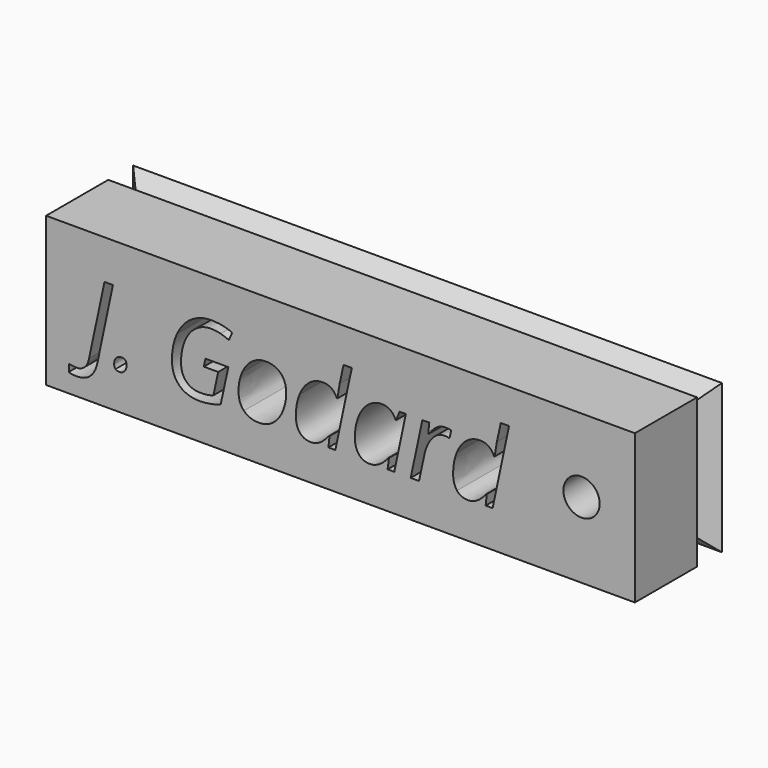
from build123d import *

# Parameters (mm, degrees)
F0_W        = 96.2526388466
F0_H        = 24.3639480323
F0_R        = 2.9624305705
F1_DEPTH    = 5.08
F2_T1_DEPTH = 50.49224719
F2_T3_DEPTH = 122.3809380044
F3_DEPTH    = 12.7


# Not quite as in the source:
# - a fillet or chamfer that OpenCascade refuses, or shapes differently, is made with other operations: its cross-section is extruded or revolved along the edge and cut away or added


with BuildPart() as f1:
    # F0 (on Front) → F1 (new body)
    with BuildSketch(Plane.XZ):
        with Locations((-21.0552643985, 29.0261851624)):
            Rectangle(F0_W, F0_H)
        with BuildLine():
            add(Edge.make_bspline(
                [(-57.832259338, 22.8351970881), (-58.0528904797, 23.0479951715), (-58.0528904797, 23.4631472607)],
                knots=[0, 0, 0, 1, 1, 1], degree=2))
            add(Edge.make_bspline(
                [(-58.0528904797, 23.4631472607), (-58.0528904797, 24.092402943), (-57.7212910123, 24.4631677019)],
                knots=[0, 0, 0, 1, 1, 1], degree=2))
            add(Edge.make_bspline(
                [(-57.7212910123, 24.4631677019), (-57.3896915448, 24.8339324608), (-56.8126562511, 24.8339324608)],
                knots=[0, 0, 0, 1, 1, 1], degree=2))
            add(Edge.make_bspline(
                [(-56.8126562511, 24.8339324608), (-56.4601686282, 24.8339324608), (-56.2447595253, 24.622439887)],
                knots=[0, 0, 0, 1, 1, 1], degree=2))
            add(Edge.make_bspline(
                [(-56.2447595253, 24.622439887), (-56.0293504225, 24.4109473133), (-56.0293504225, 23.9775180881)],
                knots=[0, 0, 0, 1, 1, 1], degree=2))
            add(Edge.make_bspline(
                [(-56.0293504225, 23.9775180881), (-56.0293504225, 23.397871775), (-56.355727851, 23.0101353898)],
                knots=[0, 0, 0, 1, 1, 1], degree=2))
            add(Edge.make_bspline(
                [(-56.355727851, 23.0101353898), (-56.6821052796, 22.6223990046), (-57.2356413985, 22.6223990046)],
                knots=[0, 0, 0, 1, 1, 1], degree=2))
            add(Edge.make_bspline(
                [(-57.2356413985, 22.6223990046), (-57.6116281963, 22.6223990046), (-57.832259338, 22.8351970881)],
                knots=[0, 0, 0, 1, 1, 1], degree=2))
        make_face(mode=Mode.SUBTRACT)
        with BuildLine():
            add(Edge.make_bspline(
                [(-60.7761837439, 22.8103924035), (-61.4211055428, 19.7189453999), (-64.2201183703, 19.7189453999)],
                knots=[0, 0, 0, 1, 1, 1], degree=2))
            add(Edge.make_bspline(
                [(-64.2201183703, 19.7189453999), (-65.076532743, 19.7189453999), (-65.4681856573, 19.9226049153)],
                knots=[0, 0, 0, 1, 1, 1], degree=2))
            Line((-65.4681856573, 19.9226049153), (-65.4185762881, 21.1210628331))
            add(Edge.make_bspline(
                [(-65.4185762881, 21.1210628331), (-64.8572071109, 20.9591796285), (-64.2357844869, 20.9591796285)],
                knots=[0, 0, 0, 1, 1, 1], degree=2))
            add(Edge.make_bspline(
                [(-64.2357844869, 20.9591796285), (-63.4211464251, 20.9591796285), (-62.8858874423, 21.4683284171)],
                knots=[0, 0, 0, 1, 1, 1], degree=2))
            add(Edge.make_bspline(
                [(-62.8858874423, 21.4683284171), (-62.3506284594, 21.9774772057), (-62.1469689439, 22.9592205109)],
                knots=[0, 0, 0, 1, 1, 1], degree=2))
            Line((-62.1469689439, 22.9592205109), (-59.6430013118, 34.7897495424))
            Line((-59.6430013118, 34.7897495424), (-58.2539389757, 34.7897495424))
            Line((-58.2539389757, 34.7897495424), (-60.7761837439, 22.8103924035))
        make_face(mode=Mode.SUBTRACT)
        with BuildLine():
            add(Edge.make_bspline(
                [(-35.5210983196, 31.1865427308), (-34.509328291, 31.9176281709), (-33.2795381401, 31.9176281709)],
                knots=[0, 0, 0, 1, 1, 1], degree=2))
            add(Edge.make_bspline(
                [(-33.2795381401, 31.9176281709), (-31.7285925994, 31.9176281709), (-30.8304019159, 30.9998548417)],
                knots=[0, 0, 0, 1, 1, 1], degree=2))
            add(Edge.make_bspline(
                [(-30.8304019159, 30.9998548417), (-29.9322112324, 30.0820815125), (-29.9322112324, 28.4736935444)],
                knots=[0, 0, 0, 1, 1, 1], degree=2))
            add(Edge.make_bspline(
                [(-29.9322112324, 28.4736935444), (-29.9322112324, 26.9410251397), (-30.5196906039, 25.5780729979)],
                knots=[0, 0, 0, 1, 1, 1], degree=2))
            add(Edge.make_bspline(
                [(-30.5196906039, 25.5780729979), (-31.1071699754, 24.2151208561), (-32.1111069457, 23.4722858287)],
                knots=[0, 0, 0, 1, 1, 1], degree=2))
            add(Edge.make_bspline(
                [(-32.1111069457, 23.4722858287), (-33.115043916, 22.7294508012), (-34.3787773195, 22.7294508012)],
                knots=[0, 0, 0, 1, 1, 1], degree=2))
            add(Edge.make_bspline(
                [(-34.3787773195, 22.7294508012), (-35.9453889768, 22.7294508012), (-36.835746602, 23.6511406595)],
                knots=[0, 0, 0, 1, 1, 1], degree=2))
            add(Edge.make_bspline(
                [(-36.835746602, 23.6511406595), (-37.7261042272, 24.5728305179), (-37.7261042272, 26.1733854277)],
                knots=[0, 0, 0, 1, 1, 1], degree=2))
            add(Edge.make_bspline(
                [(-37.7261042272, 26.1733854277), (-37.7261042272, 27.7243309683), (-37.1294862877, 29.0898941296)],
                knots=[0, 0, 0, 1, 1, 1], degree=2))
            add(Edge.make_bspline(
                [(-37.1294862877, 29.0898941296), (-36.5328683482, 30.4554572908), (-35.5210983196, 31.1865427308)],
                knots=[0, 0, 0, 1, 1, 1], degree=2))
        make_face(mode=Mode.SUBTRACT)
        with BuildLine():
            Line((-43.4024604652, 27.8705480563), (-43.133525464, 29.110782285))
            Line((-43.133525464, 29.110782285), (-39.3893236032, 29.110782285))
            Line((-39.3893236032, 29.110782285), (-40.6452239485, 23.3090971144))
            add(Edge.make_bspline(
                [(-40.6452239485, 23.3090971144), (-42.4076620628, 22.6955075486), (-44.0656594001, 22.6955075486)],
                knots=[0, 0, 0, 1, 1, 1], degree=2))
            add(Edge.make_bspline(
                [(-44.0656594001, 22.6955075486), (-46.2197504288, 22.6955075486), (-47.4142918174, 23.8756883304)],
                knots=[0, 0, 0, 1, 1, 1], degree=2))
            add(Edge.make_bspline(
                [(-47.4142918174, 23.8756883304), (-48.608833206, 25.0558691122), (-48.608833206, 27.16818383)],
                knots=[0, 0, 0, 1, 1, 1], degree=2))
            add(Edge.make_bspline(
                [(-48.608833206, 27.16818383), (-48.608833206, 29.3640511696), (-47.7811400471, 31.163043556)],
                knots=[0, 0, 0, 1, 1, 1], degree=2))
            add(Edge.make_bspline(
                [(-47.7811400471, 31.163043556), (-46.9534468882, 32.9620359423), (-45.4847484596, 33.9607508738)],
                knots=[0, 0, 0, 1, 1, 1], degree=2))
            add(Edge.make_bspline(
                [(-45.4847484596, 33.9607508738), (-44.0160500309, 34.9594658053), (-42.2275017223, 34.9594658053)],
                knots=[0, 0, 0, 1, 1, 1], degree=2))
            add(Edge.make_bspline(
                [(-42.2275017223, 34.9594658053), (-41.2744796308, 34.9594658053), (-40.4376479039, 34.796277091)],
                knots=[0, 0, 0, 1, 1, 1], degree=2))
            add(Edge.make_bspline(
                [(-40.4376479039, 34.796277091), (-39.600816177, 34.6330883767), (-38.7522348626, 34.275378715)],
                knots=[0, 0, 0, 1, 1, 1], degree=2))
            Line((-38.7522348626, 34.275378715), (-39.290104865, 33.0351444863))
            add(Edge.make_bspline(
                [(-39.290104865, 33.0351444863), (-39.9193605473, 33.3119125458), (-40.6413074193, 33.5155720612)],
                knots=[0, 0, 0, 1, 1, 1], degree=2))
            add(Edge.make_bspline(
                [(-40.6413074193, 33.5155720612), (-41.3632542914, 33.7192315767), (-42.2275017223, 33.7192315767)],
                knots=[0, 0, 0, 1, 1, 1], degree=2))
            add(Edge.make_bspline(
                [(-42.2275017223, 33.7192315767), (-43.6087310001, 33.7192315767), (-44.737996903, 32.8915384178)],
                knots=[0, 0, 0, 1, 1, 1], degree=2))
            add(Edge.make_bspline(
                [(-44.737996903, 32.8915384178), (-45.8672628059, 32.0638452589), (-46.4952129785, 30.5794807136)],
                knots=[0, 0, 0, 1, 1, 1], degree=2))
            add(Edge.make_bspline(
                [(-46.4952129785, 30.5794807136), (-47.1231631511, 29.0951161684), (-47.1231631511, 27.2569584906)],
                knots=[0, 0, 0, 1, 1, 1], degree=2))
            add(Edge.make_bspline(
                [(-47.1231631511, 27.2569584906), (-47.1231631511, 25.7086239694), (-46.2876369339, 24.8182663442)],
                knots=[0, 0, 0, 1, 1, 1], degree=2))
            add(Edge.make_bspline(
                [(-46.2876369339, 24.8182663442), (-45.4521107167, 23.927908719), (-43.9507745452, 23.927908719)],
                knots=[0, 0, 0, 1, 1, 1], degree=2))
            add(Edge.make_bspline(
                [(-43.9507745452, 23.927908719), (-42.6948742, 23.927908719), (-41.8280157497, 24.2464530893)],
                knots=[0, 0, 0, 1, 1, 1], degree=2))
            Line((-41.8280157497, 24.2464530893), (-41.0447099211, 27.8705480563))
            Line((-41.0447099211, 27.8705480563), (-43.4024604652, 27.8705480563))
        make_face(mode=Mode.SUBTRACT)
        with BuildLine():
            add(Edge.make_bspline(
                [(-16.5259319757, 31.1421554005), (-15.5063288888, 31.96723754), (-14.289593835, 31.96723754)],
                knots=[0, 0, 0, 1, 1, 1], degree=2))
            add(Edge.make_bspline(
                [(-14.289593835, 31.96723754), (-13.540231259, 31.96723754), (-12.9527518875, 31.5625295286)],
                knots=[0, 0, 0, 1, 1, 1], degree=2))
            add(Edge.make_bspline(
                [(-12.9527518875, 31.5625295286), (-12.365272516, 31.1578215171), (-12.0388950874, 30.4006258828)],
                knots=[0, 0, 0, 1, 1, 1], degree=2))
            Line((-12.0388950874, 30.4006258828), (-11.9475094074, 30.4006258828))
            Line((-11.9475094074, 30.4006258828), (-11.4018063468, 31.802743316))
            Line((-11.4018063468, 31.802743316), (-10.3652316336, 31.802743316))
            Line((-10.3652316336, 31.802743316), (-12.2660537777, 22.8600017726))
            Line((-12.2660537777, 22.8600017726), (-13.3522378601, 22.8600017726))
            Line((-13.3522378601, 22.8600017726), (-13.1381342669, 24.5649974596))
            Line((-13.1381342669, 24.5649974596), (-13.2034097527, 24.5649974596))
            add(Edge.make_bspline(
                [(-13.2034097527, 24.5649974596), (-14.6655806327, 22.6955075486), (-16.2818016591, 22.6955075486)],
                knots=[0, 0, 0, 1, 1, 1], degree=2))
            add(Edge.make_bspline(
                [(-16.2818016591, 22.6955075486), (-17.4149840912, 22.6955075486), (-18.0599058901, 23.5036180618)],
                knots=[0, 0, 0, 1, 1, 1], degree=2))
            add(Edge.make_bspline(
                [(-18.0599058901, 23.5036180618), (-18.704827689, 24.311728575), (-18.704827689, 25.7164570277)],
                knots=[0, 0, 0, 1, 1, 1], degree=2))
            add(Edge.make_bspline(
                [(-18.704827689, 25.7164570277), (-18.704827689, 27.4136196563), (-18.1251813758, 28.8653464587)],
                knots=[0, 0, 0, 1, 1, 1], degree=2))
            add(Edge.make_bspline(
                [(-18.1251813758, 28.8653464587), (-17.5455350626, 30.3170732611), (-16.5259319757, 31.1421554005)],
                knots=[0, 0, 0, 1, 1, 1], degree=2))
        make_face(mode=Mode.SUBTRACT)
        with BuildLine():
            add(Edge.make_bspline(
                [(-4.8612026779, 31.7831606703), (-4.4408285499, 31.96723754), (-3.9264577224, 31.96723754)],
                knots=[0, 0, 0, 1, 1, 1], degree=2))
            add(Edge.make_bspline(
                [(-3.9264577224, 31.96723754), (-3.3624775258, 31.96723754), (-2.9473254367, 31.8523526851)],
                knots=[0, 0, 0, 1, 1, 1], degree=2))
            Line((-2.9473254367, 31.8523526851), (-3.2397596127, 30.6277845731))
            add(Edge.make_bspline(
                [(-3.2397596127, 30.6277845731), (-3.6731888378, 30.7348363696), (-4.0987850047, 30.7348363696)],
                knots=[0, 0, 0, 1, 1, 1], degree=2))
            add(Edge.make_bspline(
                [(-4.0987850047, 30.7348363696), (-4.8403145225, 30.7348363696), (-5.4891528505, 30.2452702268)],
                knots=[0, 0, 0, 1, 1, 1], degree=2))
            add(Edge.make_bspline(
                [(-5.4891528505, 30.2452702268), (-6.1379911785, 29.7557040839), (-6.6236407923, 28.8862346141)],
                knots=[0, 0, 0, 1, 1, 1], degree=2))
            add(Edge.make_bspline(
                [(-6.6236407923, 28.8862346141), (-7.109290406, 28.0167651444), (-7.3364490963, 26.9566912563)],
                knots=[0, 0, 0, 1, 1, 1], degree=2))
            Line((-7.3364490963, 26.9566912563), (-8.2111406049, 22.8600017726))
            Line((-8.2111406049, 22.8600017726), (-9.581925805, 22.8600017726))
            Line((-9.581925805, 22.8600017726), (-7.6706595832, 31.802743316))
            Line((-7.6706595832, 31.802743316), (-6.5374771511, 31.802743316))
            Line((-6.5374771511, 31.802743316), (-6.7176374917, 30.1473569982))
            Line((-6.7176374917, 30.1473569982), (-6.63408487, 30.1473569982))
            add(Edge.make_bspline(
                [(-6.63408487, 30.1473569982), (-6.0466054985, 30.9228297685), (-5.6640911522, 31.2609567845)],
                knots=[0, 0, 0, 1, 1, 1], degree=2))
            add(Edge.make_bspline(
                [(-5.6640911522, 31.2609567845), (-5.2815768059, 31.5990838006), (-4.8612026779, 31.7831606703)],
                knots=[0, 0, 0, 1, 1, 1], degree=2))
        make_face(mode=Mode.SUBTRACT)
        with BuildLine():
            add(Edge.make_bspline(
                [(-26.1749542745, 31.1578215171), (-25.1749338333, 31.948960404), (-23.9346996047, 31.948960404)],
                knots=[0, 0, 0, 1, 1, 1], degree=2))
            add(Edge.make_bspline(
                [(-23.9346996047, 31.948960404), (-22.3524218309, 31.948960404), (-21.6422245463, 30.4006258828)],
                knots=[0, 0, 0, 1, 1, 1], degree=2))
            Line((-21.6422245463, 30.4006258828), (-21.561282944, 30.4006258828))
            add(Edge.make_bspline(
                [(-21.561282944, 30.4006258828), (-21.4228989143, 31.6643592863), (-21.1931292045, 32.6356585138)],
                knots=[0, 0, 0, 1, 1, 1], degree=2))
            Line((-21.1931292045, 32.6356585138), (-20.5560404639, 35.5573892545))
            Line((-20.5560404639, 35.5573892545), (-19.2035323998, 35.5573892545))
            Line((-19.2035323998, 35.5573892545), (-21.8954934308, 22.8600017726))
            Line((-21.8954934308, 22.8600017726), (-23.0286758629, 22.8600017726))
            Line((-23.0286758629, 22.8600017726), (-22.8485155223, 24.5649974596))
            Line((-22.8485155223, 24.5649974596), (-22.913791008, 24.5649974596))
            add(Edge.make_bspline(
                [(-22.913791008, 24.5649974596), (-23.7388731475, 23.5466998824), (-24.4569034904, 23.1211037155)],
                knots=[0, 0, 0, 1, 1, 1], degree=2))
            add(Edge.make_bspline(
                [(-24.4569034904, 23.1211037155), (-25.1749338333, 22.6955075486), (-25.9425735454, 22.6955075486)],
                knots=[0, 0, 0, 1, 1, 1], degree=2))
            add(Edge.make_bspline(
                [(-25.9425735454, 22.6955075486), (-27.0757559774, 22.6955075486), (-27.712844718, 23.4957850035)],
                knots=[0, 0, 0, 1, 1, 1], degree=2))
            add(Edge.make_bspline(
                [(-27.712844718, 23.4957850035), (-28.3499334586, 24.2960624584), (-28.3499334586, 25.7164570277)],
                knots=[0, 0, 0, 1, 1, 1], degree=2))
            add(Edge.make_bspline(
                [(-28.3499334586, 25.7164570277), (-28.3499334586, 27.4632290255), (-27.7624540872, 28.9149558278)],
                knots=[0, 0, 0, 1, 1, 1], degree=2))
            add(Edge.make_bspline(
                [(-27.7624540872, 28.9149558278), (-27.1749747157, 30.3666826302), (-26.1749542745, 31.1578215171)],
                knots=[0, 0, 0, 1, 1, 1], degree=2))
        make_face(mode=Mode.SUBTRACT)
        with BuildLine():
            add(Edge.make_bspline(
                [(-0.4720790182, 31.1578215171), (0.527941423, 31.948960404), (1.7681756516, 31.948960404)],
                knots=[0, 0, 0, 1, 1, 1], degree=2))
            add(Edge.make_bspline(
                [(1.7681756516, 31.948960404), (3.3504534254, 31.948960404), (4.06065071, 30.4006258828)],
                knots=[0, 0, 0, 1, 1, 1], degree=2))
            Line((4.06065071, 30.4006258828), (4.1415923123, 30.4006258828))
            add(Edge.make_bspline(
                [(4.1415923123, 30.4006258828), (4.279976342, 31.6643592863), (4.5097460518, 32.6356585138)],
                knots=[0, 0, 0, 1, 1, 1], degree=2))
            Line((4.5097460518, 32.6356585138), (5.1468347924, 35.5573892545))
            Line((5.1468347924, 35.5573892545), (6.4993428564, 35.5573892545))
            Line((6.4993428564, 35.5573892545), (3.8073818254, 22.8600017726))
            Line((3.8073818254, 22.8600017726), (2.6741993934, 22.8600017726))
            Line((2.6741993934, 22.8600017726), (2.8543597339, 24.5649974596))
            Line((2.8543597339, 24.5649974596), (2.7890842482, 24.5649974596))
            add(Edge.make_bspline(
                [(2.7890842482, 24.5649974596), (1.9640021088, 23.5466998824), (1.2459717659, 23.1211037155)],
                knots=[0, 0, 0, 1, 1, 1], degree=2))
            add(Edge.make_bspline(
                [(1.2459717659, 23.1211037155), (0.527941423, 22.6955075486), (-0.2396982891, 22.6955075486)],
                knots=[0, 0, 0, 1, 1, 1], degree=2))
            add(Edge.make_bspline(
                [(-0.2396982891, 22.6955075486), (-1.3728807211, 22.6955075486), (-2.0099694617, 23.4957850035)],
                knots=[0, 0, 0, 1, 1, 1], degree=2))
            add(Edge.make_bspline(
                [(-2.0099694617, 23.4957850035), (-2.6470582024, 24.2960624584), (-2.6470582024, 25.7164570277)],
                knots=[0, 0, 0, 1, 1, 1], degree=2))
            add(Edge.make_bspline(
                [(-2.6470582024, 25.7164570277), (-2.6470582024, 27.4632290255), (-2.0595788309, 28.9149558278)],
                knots=[0, 0, 0, 1, 1, 1], degree=2))
            add(Edge.make_bspline(
                [(-2.0595788309, 28.9149558278), (-1.4720994594, 30.3666826302), (-0.4720790182, 31.1578215171)],
                knots=[0, 0, 0, 1, 1, 1], degree=2))
        make_face(mode=Mode.SUBTRACT)
        with Locations((18.3481574059, 29.1765797883)):
            Circle(F0_R, mode=Mode.SUBTRACT)
    extrude(amount=-F1_DEPTH)

    # F2: chamfer of 5.08 on 4 edges, made by hand

    # F2_s2 → F2_t1 (cut)
    with BuildSketch(Plane.XY.offset(3.7800615674)):
        Polygon((27.0710550249, 5.08), (21.9910550249, 0), (27.0710550249, 0), align=None)
        Polygon((-69.1815838218, 5.08), (-64.1015838218, 0), (-69.1815838218, 0), align=None)
    extrude(amount=F2_T1_DEPTH, mode=Mode.SUBTRACT)

    # F2_s4 → F2_t3 (cut)
    with BuildSketch(Plane.YZ.offset(-82.2457334006)):
        Polygon((5.08, 16.8442111462), (0, 21.9242111462), (0, 16.8442111462), align=None)
        Polygon((5.08, 41.2081591785), (0, 36.1281591785), (0, 41.2081591785), align=None)
    extrude(amount=F2_T3_DEPTH, mode=Mode.SUBTRACT)

    # F0 (on Front) → F3 (join)
    with BuildSketch(Plane.XZ):
        with Locations((-21.0552643985, 29.0261851624)):
            Rectangle(F0_W, F0_H)
        with BuildLine():
            add(Edge.make_bspline(
                [(-57.832259338, 22.8351970881), (-58.0528904797, 23.0479951715), (-58.0528904797, 23.4631472607)],
                knots=[0, 0, 0, 1, 1, 1], degree=2))
            add(Edge.make_bspline(
                [(-58.0528904797, 23.4631472607), (-58.0528904797, 24.092402943), (-57.7212910123, 24.4631677019)],
                knots=[0, 0, 0, 1, 1, 1], degree=2))
            add(Edge.make_bspline(
                [(-57.7212910123, 24.4631677019), (-57.3896915448, 24.8339324608), (-56.8126562511, 24.8339324608)],
                knots=[0, 0, 0, 1, 1, 1], degree=2))
            add(Edge.make_bspline(
                [(-56.8126562511, 24.8339324608), (-56.4601686282, 24.8339324608), (-56.2447595253, 24.622439887)],
                knots=[0, 0, 0, 1, 1, 1], degree=2))
            add(Edge.make_bspline(
                [(-56.2447595253, 24.622439887), (-56.0293504225, 24.4109473133), (-56.0293504225, 23.9775180881)],
                knots=[0, 0, 0, 1, 1, 1], degree=2))
            add(Edge.make_bspline(
                [(-56.0293504225, 23.9775180881), (-56.0293504225, 23.397871775), (-56.355727851, 23.0101353898)],
                knots=[0, 0, 0, 1, 1, 1], degree=2))
            add(Edge.make_bspline(
                [(-56.355727851, 23.0101353898), (-56.6821052796, 22.6223990046), (-57.2356413985, 22.6223990046)],
                knots=[0, 0, 0, 1, 1, 1], degree=2))
            add(Edge.make_bspline(
                [(-57.2356413985, 22.6223990046), (-57.6116281963, 22.6223990046), (-57.832259338, 22.8351970881)],
                knots=[0, 0, 0, 1, 1, 1], degree=2))
        make_face(mode=Mode.SUBTRACT)
        with BuildLine():
            add(Edge.make_bspline(
                [(-60.7761837439, 22.8103924035), (-61.4211055428, 19.7189453999), (-64.2201183703, 19.7189453999)],
                knots=[0, 0, 0, 1, 1, 1], degree=2))
            add(Edge.make_bspline(
                [(-64.2201183703, 19.7189453999), (-65.076532743, 19.7189453999), (-65.4681856573, 19.9226049153)],
                knots=[0, 0, 0, 1, 1, 1], degree=2))
            Line((-65.4681856573, 19.9226049153), (-65.4185762881, 21.1210628331))
            add(Edge.make_bspline(
                [(-65.4185762881, 21.1210628331), (-64.8572071109, 20.9591796285), (-64.2357844869, 20.9591796285)],
                knots=[0, 0, 0, 1, 1, 1], degree=2))
            add(Edge.make_bspline(
                [(-64.2357844869, 20.9591796285), (-63.4211464251, 20.9591796285), (-62.8858874423, 21.4683284171)],
                knots=[0, 0, 0, 1, 1, 1], degree=2))
            add(Edge.make_bspline(
                [(-62.8858874423, 21.4683284171), (-62.3506284594, 21.9774772057), (-62.1469689439, 22.9592205109)],
                knots=[0, 0, 0, 1, 1, 1], degree=2))
            Line((-62.1469689439, 22.9592205109), (-59.6430013118, 34.7897495424))
            Line((-59.6430013118, 34.7897495424), (-58.2539389757, 34.7897495424))
            Line((-58.2539389757, 34.7897495424), (-60.7761837439, 22.8103924035))
        make_face(mode=Mode.SUBTRACT)
        with BuildLine():
            add(Edge.make_bspline(
                [(-35.5210983196, 31.1865427308), (-34.509328291, 31.9176281709), (-33.2795381401, 31.9176281709)],
                knots=[0, 0, 0, 1, 1, 1], degree=2))
            add(Edge.make_bspline(
                [(-33.2795381401, 31.9176281709), (-31.7285925994, 31.9176281709), (-30.8304019159, 30.9998548417)],
                knots=[0, 0, 0, 1, 1, 1], degree=2))
            add(Edge.make_bspline(
                [(-30.8304019159, 30.9998548417), (-29.9322112324, 30.0820815125), (-29.9322112324, 28.4736935444)],
                knots=[0, 0, 0, 1, 1, 1], degree=2))
            add(Edge.make_bspline(
                [(-29.9322112324, 28.4736935444), (-29.9322112324, 26.9410251397), (-30.5196906039, 25.5780729979)],
                knots=[0, 0, 0, 1, 1, 1], degree=2))
            add(Edge.make_bspline(
                [(-30.5196906039, 25.5780729979), (-31.1071699754, 24.2151208561), (-32.1111069457, 23.4722858287)],
                knots=[0, 0, 0, 1, 1, 1], degree=2))
            add(Edge.make_bspline(
                [(-32.1111069457, 23.4722858287), (-33.115043916, 22.7294508012), (-34.3787773195, 22.7294508012)],
                knots=[0, 0, 0, 1, 1, 1], degree=2))
            add(Edge.make_bspline(
                [(-34.3787773195, 22.7294508012), (-35.9453889768, 22.7294508012), (-36.835746602, 23.6511406595)],
                knots=[0, 0, 0, 1, 1, 1], degree=2))
            add(Edge.make_bspline(
                [(-36.835746602, 23.6511406595), (-37.7261042272, 24.5728305179), (-37.7261042272, 26.1733854277)],
                knots=[0, 0, 0, 1, 1, 1], degree=2))
            add(Edge.make_bspline(
                [(-37.7261042272, 26.1733854277), (-37.7261042272, 27.7243309683), (-37.1294862877, 29.0898941296)],
                knots=[0, 0, 0, 1, 1, 1], degree=2))
            add(Edge.make_bspline(
                [(-37.1294862877, 29.0898941296), (-36.5328683482, 30.4554572908), (-35.5210983196, 31.1865427308)],
                knots=[0, 0, 0, 1, 1, 1], degree=2))
        make_face(mode=Mode.SUBTRACT)
        with BuildLine():
            Line((-43.4024604652, 27.8705480563), (-43.133525464, 29.110782285))
            Line((-43.133525464, 29.110782285), (-39.3893236032, 29.110782285))
            Line((-39.3893236032, 29.110782285), (-40.6452239485, 23.3090971144))
            add(Edge.make_bspline(
                [(-40.6452239485, 23.3090971144), (-42.4076620628, 22.6955075486), (-44.0656594001, 22.6955075486)],
                knots=[0, 0, 0, 1, 1, 1], degree=2))
            add(Edge.make_bspline(
                [(-44.0656594001, 22.6955075486), (-46.2197504288, 22.6955075486), (-47.4142918174, 23.8756883304)],
                knots=[0, 0, 0, 1, 1, 1], degree=2))
            add(Edge.make_bspline(
                [(-47.4142918174, 23.8756883304), (-48.608833206, 25.0558691122), (-48.608833206, 27.16818383)],
                knots=[0, 0, 0, 1, 1, 1], degree=2))
            add(Edge.make_bspline(
                [(-48.608833206, 27.16818383), (-48.608833206, 29.3640511696), (-47.7811400471, 31.163043556)],
                knots=[0, 0, 0, 1, 1, 1], degree=2))
            add(Edge.make_bspline(
                [(-47.7811400471, 31.163043556), (-46.9534468882, 32.9620359423), (-45.4847484596, 33.9607508738)],
                knots=[0, 0, 0, 1, 1, 1], degree=2))
            add(Edge.make_bspline(
                [(-45.4847484596, 33.9607508738), (-44.0160500309, 34.9594658053), (-42.2275017223, 34.9594658053)],
                knots=[0, 0, 0, 1, 1, 1], degree=2))
            add(Edge.make_bspline(
                [(-42.2275017223, 34.9594658053), (-41.2744796308, 34.9594658053), (-40.4376479039, 34.796277091)],
                knots=[0, 0, 0, 1, 1, 1], degree=2))
            add(Edge.make_bspline(
                [(-40.4376479039, 34.796277091), (-39.600816177, 34.6330883767), (-38.7522348626, 34.275378715)],
                knots=[0, 0, 0, 1, 1, 1], degree=2))
            Line((-38.7522348626, 34.275378715), (-39.290104865, 33.0351444863))
            add(Edge.make_bspline(
                [(-39.290104865, 33.0351444863), (-39.9193605473, 33.3119125458), (-40.6413074193, 33.5155720612)],
                knots=[0, 0, 0, 1, 1, 1], degree=2))
            add(Edge.make_bspline(
                [(-40.6413074193, 33.5155720612), (-41.3632542914, 33.7192315767), (-42.2275017223, 33.7192315767)],
                knots=[0, 0, 0, 1, 1, 1], degree=2))
            add(Edge.make_bspline(
                [(-42.2275017223, 33.7192315767), (-43.6087310001, 33.7192315767), (-44.737996903, 32.8915384178)],
                knots=[0, 0, 0, 1, 1, 1], degree=2))
            add(Edge.make_bspline(
                [(-44.737996903, 32.8915384178), (-45.8672628059, 32.0638452589), (-46.4952129785, 30.5794807136)],
                knots=[0, 0, 0, 1, 1, 1], degree=2))
            add(Edge.make_bspline(
                [(-46.4952129785, 30.5794807136), (-47.1231631511, 29.0951161684), (-47.1231631511, 27.2569584906)],
                knots=[0, 0, 0, 1, 1, 1], degree=2))
            add(Edge.make_bspline(
                [(-47.1231631511, 27.2569584906), (-47.1231631511, 25.7086239694), (-46.2876369339, 24.8182663442)],
                knots=[0, 0, 0, 1, 1, 1], degree=2))
            add(Edge.make_bspline(
                [(-46.2876369339, 24.8182663442), (-45.4521107167, 23.927908719), (-43.9507745452, 23.927908719)],
                knots=[0, 0, 0, 1, 1, 1], degree=2))
            add(Edge.make_bspline(
                [(-43.9507745452, 23.927908719), (-42.6948742, 23.927908719), (-41.8280157497, 24.2464530893)],
                knots=[0, 0, 0, 1, 1, 1], degree=2))
            Line((-41.8280157497, 24.2464530893), (-41.0447099211, 27.8705480563))
            Line((-41.0447099211, 27.8705480563), (-43.4024604652, 27.8705480563))
        make_face(mode=Mode.SUBTRACT)
        with BuildLine():
            add(Edge.make_bspline(
                [(-16.5259319757, 31.1421554005), (-15.5063288888, 31.96723754), (-14.289593835, 31.96723754)],
                knots=[0, 0, 0, 1, 1, 1], degree=2))
            add(Edge.make_bspline(
                [(-14.289593835, 31.96723754), (-13.540231259, 31.96723754), (-12.9527518875, 31.5625295286)],
                knots=[0, 0, 0, 1, 1, 1], degree=2))
            add(Edge.make_bspline(
                [(-12.9527518875, 31.5625295286), (-12.365272516, 31.1578215171), (-12.0388950874, 30.4006258828)],
                knots=[0, 0, 0, 1, 1, 1], degree=2))
            Line((-12.0388950874, 30.4006258828), (-11.9475094074, 30.4006258828))
            Line((-11.9475094074, 30.4006258828), (-11.4018063468, 31.802743316))
            Line((-11.4018063468, 31.802743316), (-10.3652316336, 31.802743316))
            Line((-10.3652316336, 31.802743316), (-12.2660537777, 22.8600017726))
            Line((-12.2660537777, 22.8600017726), (-13.3522378601, 22.8600017726))
            Line((-13.3522378601, 22.8600017726), (-13.1381342669, 24.5649974596))
            Line((-13.1381342669, 24.5649974596), (-13.2034097527, 24.5649974596))
            add(Edge.make_bspline(
                [(-13.2034097527, 24.5649974596), (-14.6655806327, 22.6955075486), (-16.2818016591, 22.6955075486)],
                knots=[0, 0, 0, 1, 1, 1], degree=2))
            add(Edge.make_bspline(
                [(-16.2818016591, 22.6955075486), (-17.4149840912, 22.6955075486), (-18.0599058901, 23.5036180618)],
                knots=[0, 0, 0, 1, 1, 1], degree=2))
            add(Edge.make_bspline(
                [(-18.0599058901, 23.5036180618), (-18.704827689, 24.311728575), (-18.704827689, 25.7164570277)],
                knots=[0, 0, 0, 1, 1, 1], degree=2))
            add(Edge.make_bspline(
                [(-18.704827689, 25.7164570277), (-18.704827689, 27.4136196563), (-18.1251813758, 28.8653464587)],
                knots=[0, 0, 0, 1, 1, 1], degree=2))
            add(Edge.make_bspline(
                [(-18.1251813758, 28.8653464587), (-17.5455350626, 30.3170732611), (-16.5259319757, 31.1421554005)],
                knots=[0, 0, 0, 1, 1, 1], degree=2))
        make_face(mode=Mode.SUBTRACT)
        with BuildLine():
            add(Edge.make_bspline(
                [(-4.8612026779, 31.7831606703), (-4.4408285499, 31.96723754), (-3.9264577224, 31.96723754)],
                knots=[0, 0, 0, 1, 1, 1], degree=2))
            add(Edge.make_bspline(
                [(-3.9264577224, 31.96723754), (-3.3624775258, 31.96723754), (-2.9473254367, 31.8523526851)],
                knots=[0, 0, 0, 1, 1, 1], degree=2))
            Line((-2.9473254367, 31.8523526851), (-3.2397596127, 30.6277845731))
            add(Edge.make_bspline(
                [(-3.2397596127, 30.6277845731), (-3.6731888378, 30.7348363696), (-4.0987850047, 30.7348363696)],
                knots=[0, 0, 0, 1, 1, 1], degree=2))
            add(Edge.make_bspline(
                [(-4.0987850047, 30.7348363696), (-4.8403145225, 30.7348363696), (-5.4891528505, 30.2452702268)],
                knots=[0, 0, 0, 1, 1, 1], degree=2))
            add(Edge.make_bspline(
                [(-5.4891528505, 30.2452702268), (-6.1379911785, 29.7557040839), (-6.6236407923, 28.8862346141)],
                knots=[0, 0, 0, 1, 1, 1], degree=2))
            add(Edge.make_bspline(
                [(-6.6236407923, 28.8862346141), (-7.109290406, 28.0167651444), (-7.3364490963, 26.9566912563)],
                knots=[0, 0, 0, 1, 1, 1], degree=2))
            Line((-7.3364490963, 26.9566912563), (-8.2111406049, 22.8600017726))
            Line((-8.2111406049, 22.8600017726), (-9.581925805, 22.8600017726))
            Line((-9.581925805, 22.8600017726), (-7.6706595832, 31.802743316))
            Line((-7.6706595832, 31.802743316), (-6.5374771511, 31.802743316))
            Line((-6.5374771511, 31.802743316), (-6.7176374917, 30.1473569982))
            Line((-6.7176374917, 30.1473569982), (-6.63408487, 30.1473569982))
            add(Edge.make_bspline(
                [(-6.63408487, 30.1473569982), (-6.0466054985, 30.9228297685), (-5.6640911522, 31.2609567845)],
                knots=[0, 0, 0, 1, 1, 1], degree=2))
            add(Edge.make_bspline(
                [(-5.6640911522, 31.2609567845), (-5.2815768059, 31.5990838006), (-4.8612026779, 31.7831606703)],
                knots=[0, 0, 0, 1, 1, 1], degree=2))
        make_face(mode=Mode.SUBTRACT)
        with BuildLine():
            add(Edge.make_bspline(
                [(-26.1749542745, 31.1578215171), (-25.1749338333, 31.948960404), (-23.9346996047, 31.948960404)],
                knots=[0, 0, 0, 1, 1, 1], degree=2))
            add(Edge.make_bspline(
                [(-23.9346996047, 31.948960404), (-22.3524218309, 31.948960404), (-21.6422245463, 30.4006258828)],
                knots=[0, 0, 0, 1, 1, 1], degree=2))
            Line((-21.6422245463, 30.4006258828), (-21.561282944, 30.4006258828))
            add(Edge.make_bspline(
                [(-21.561282944, 30.4006258828), (-21.4228989143, 31.6643592863), (-21.1931292045, 32.6356585138)],
                knots=[0, 0, 0, 1, 1, 1], degree=2))
            Line((-21.1931292045, 32.6356585138), (-20.5560404639, 35.5573892545))
            Line((-20.5560404639, 35.5573892545), (-19.2035323998, 35.5573892545))
            Line((-19.2035323998, 35.5573892545), (-21.8954934308, 22.8600017726))
            Line((-21.8954934308, 22.8600017726), (-23.0286758629, 22.8600017726))
            Line((-23.0286758629, 22.8600017726), (-22.8485155223, 24.5649974596))
            Line((-22.8485155223, 24.5649974596), (-22.913791008, 24.5649974596))
            add(Edge.make_bspline(
                [(-22.913791008, 24.5649974596), (-23.7388731475, 23.5466998824), (-24.4569034904, 23.1211037155)],
                knots=[0, 0, 0, 1, 1, 1], degree=2))
            add(Edge.make_bspline(
                [(-24.4569034904, 23.1211037155), (-25.1749338333, 22.6955075486), (-25.9425735454, 22.6955075486)],
                knots=[0, 0, 0, 1, 1, 1], degree=2))
            add(Edge.make_bspline(
                [(-25.9425735454, 22.6955075486), (-27.0757559774, 22.6955075486), (-27.712844718, 23.4957850035)],
                knots=[0, 0, 0, 1, 1, 1], degree=2))
            add(Edge.make_bspline(
                [(-27.712844718, 23.4957850035), (-28.3499334586, 24.2960624584), (-28.3499334586, 25.7164570277)],
                knots=[0, 0, 0, 1, 1, 1], degree=2))
            add(Edge.make_bspline(
                [(-28.3499334586, 25.7164570277), (-28.3499334586, 27.4632290255), (-27.7624540872, 28.9149558278)],
                knots=[0, 0, 0, 1, 1, 1], degree=2))
            add(Edge.make_bspline(
                [(-27.7624540872, 28.9149558278), (-27.1749747157, 30.3666826302), (-26.1749542745, 31.1578215171)],
                knots=[0, 0, 0, 1, 1, 1], degree=2))
        make_face(mode=Mode.SUBTRACT)
        with BuildLine():
            add(Edge.make_bspline(
                [(-0.4720790182, 31.1578215171), (0.527941423, 31.948960404), (1.7681756516, 31.948960404)],
                knots=[0, 0, 0, 1, 1, 1], degree=2))
            add(Edge.make_bspline(
                [(1.7681756516, 31.948960404), (3.3504534254, 31.948960404), (4.06065071, 30.4006258828)],
                knots=[0, 0, 0, 1, 1, 1], degree=2))
            Line((4.06065071, 30.4006258828), (4.1415923123, 30.4006258828))
            add(Edge.make_bspline(
                [(4.1415923123, 30.4006258828), (4.279976342, 31.6643592863), (4.5097460518, 32.6356585138)],
                knots=[0, 0, 0, 1, 1, 1], degree=2))
            Line((4.5097460518, 32.6356585138), (5.1468347924, 35.5573892545))
            Line((5.1468347924, 35.5573892545), (6.4993428564, 35.5573892545))
            Line((6.4993428564, 35.5573892545), (3.8073818254, 22.8600017726))
            Line((3.8073818254, 22.8600017726), (2.6741993934, 22.8600017726))
            Line((2.6741993934, 22.8600017726), (2.8543597339, 24.5649974596))
            Line((2.8543597339, 24.5649974596), (2.7890842482, 24.5649974596))
            add(Edge.make_bspline(
                [(2.7890842482, 24.5649974596), (1.9640021088, 23.5466998824), (1.2459717659, 23.1211037155)],
                knots=[0, 0, 0, 1, 1, 1], degree=2))
            add(Edge.make_bspline(
                [(1.2459717659, 23.1211037155), (0.527941423, 22.6955075486), (-0.2396982891, 22.6955075486)],
                knots=[0, 0, 0, 1, 1, 1], degree=2))
            add(Edge.make_bspline(
                [(-0.2396982891, 22.6955075486), (-1.3728807211, 22.6955075486), (-2.0099694617, 23.4957850035)],
                knots=[0, 0, 0, 1, 1, 1], degree=2))
            add(Edge.make_bspline(
                [(-2.0099694617, 23.4957850035), (-2.6470582024, 24.2960624584), (-2.6470582024, 25.7164570277)],
                knots=[0, 0, 0, 1, 1, 1], degree=2))
            add(Edge.make_bspline(
                [(-2.6470582024, 25.7164570277), (-2.6470582024, 27.4632290255), (-2.0595788309, 28.9149558278)],
                knots=[0, 0, 0, 1, 1, 1], degree=2))
            add(Edge.make_bspline(
                [(-2.0595788309, 28.9149558278), (-1.4720994594, 30.3666826302), (-0.4720790182, 31.1578215171)],
                knots=[0, 0, 0, 1, 1, 1], degree=2))
        make_face(mode=Mode.SUBTRACT)
        with Locations((18.3481574059, 29.1765797883)):
            Circle(F0_R, mode=Mode.SUBTRACT)
    extrude(amount=F3_DEPTH)


solid = f1.part
